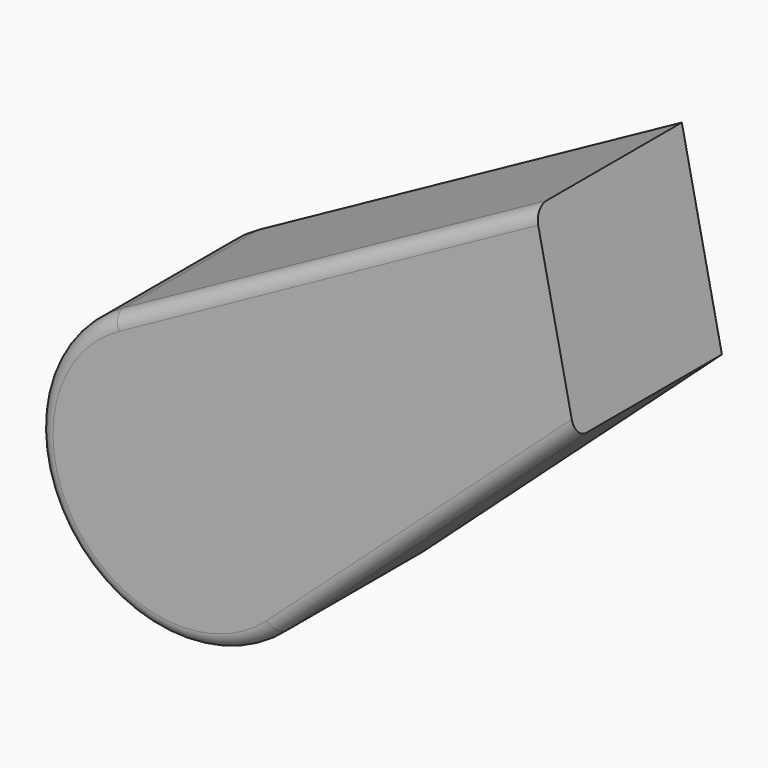
from build123d import *

# Parameters (mm, degrees)
F1_DEPTH = 25.4
F2_R     = 2
F3_T     = 2


# Not quite as in the source:
# - a shell that OpenCascade refuses in one call is made with other operations: the cavity is built on its own and cut out


with BuildPart() as f1:
    # F0 (on Front) → F1 (new body)
    with BuildSketch(Plane.XZ):
        with BuildLine():
            Line((-51.5017161099, 61.5344954622), (-110.0323972047, 29.4426782099))
            ThreePointArc((-110.0323972047, 29.4426782099), (-116.6082312435, 0.741485542), (-87.3347394228, -2.4306951723))
            Line((-87.3347394228, -2.4306951723), (-45.9517985582, 35.0605621934))
            Line((-45.9517985582, 35.0605621934), (-51.5017161099, 61.5344954622))
        make_face()
    extrude(amount=F1_DEPTH)

    # F2
    f2_edges = [f1.edges().sort_by_distance(p)[0] for p in [
        (-80.767057, -25.4, 45.488587),
    ]]
    fillet(f2_edges, radius=F2_R)

    # F3: shell of thickness 2, made by hand


with BuildPart() as f3_core1:
    # F3_t2: copy of F1
    add(f1.part)

    # the walls: a layer under each face that stays
    f3_faces = [f3_core1.faces().sort_by_distance(p)[0] for p in [
        (-66.6432689905, -11.7, 16.3149335105),
        (-116.6082312435, -11.7, 0.741485542),
        (-48.7267573341, -12.7, 48.2975288278),
        (-80.7670566573, -11.7, 45.488586836),
        (-82.3442492315, -25.4, 26.9788079772),
    ]]
    thicken(f3_faces, amount=-F3_T, mode=Mode.SUBTRACT)


with BuildPart() as f1_1:
    add(f1.part)

    # what is left inside the walls is the cavity
    f3_cavity = [f3_core1.part.solids().sort_by_distance(p)[0] for p in [
        (-83.202908, -0.02, 15.807193),
    ]]
    add(f3_cavity, mode=Mode.SUBTRACT)


solid = f1_1.part
